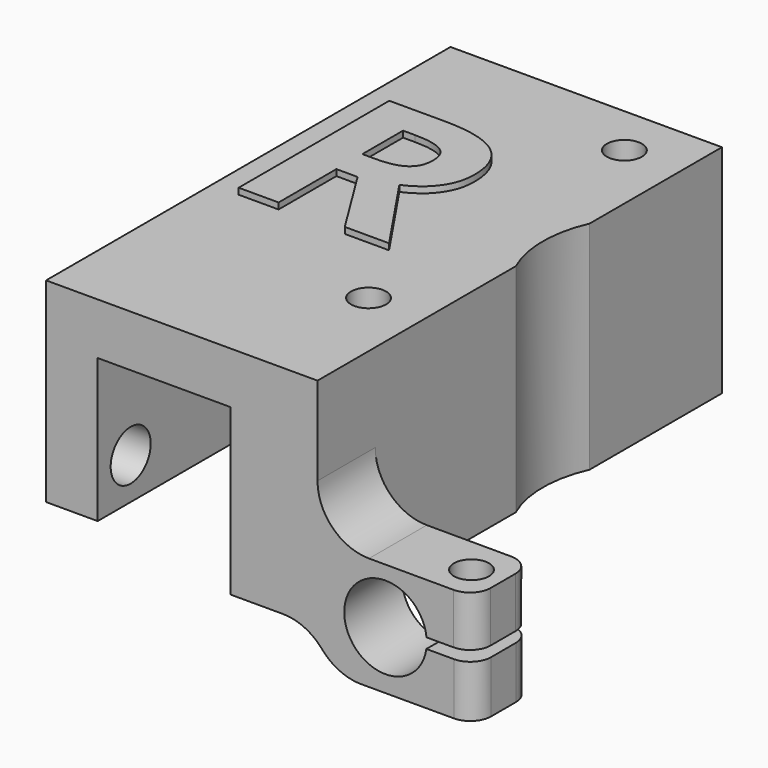
from build123d import *

# Parameters (mm, degrees)
F1_DEPTH      = 7
F2_DEPTH      = 42
F3_R          = 1.7
F3_R_2        = 11
F4_DEPTH      = 21.001
F5_R          = 4
F6_DEPTH      = 10
F7_DEPTH      = 21.001
F8_R          = 1.4
F9_DEPTH      = 11.021861364
F8_R_2        = 1.7
F10_DEPTH     = 4.9110969969
F11_R         = 5
F12_R         = 5
F13_R         = 5
F14_R         = 2
F15_R         = 2.2
F15_R_2       = 2.4255023423
F16_DEPTH     = 6
F17_TEXT_SIZE = 25.5631890872
F18_DEPTH     = 0.6


# Not quite as in the source:
# - a feature names something its author has since deleted; it is built from what else it names
# - Text() gives the source's letters only with a copy of the font that has no kerning and outlines rounded to 1/6400 em; it was checked with that copy


with BuildPart() as f1:
    # F0 (on Front) → F1 (new body)
    with BuildSketch(Plane.XZ):
        Polygon((-18.6721007523, 29.8099789735), (-18.6721007523, 10.8925135386), (-13.6721007523, 10.8925135386), (-13.6721007523, 24.8099789735), (-0.7721007523, 24.8099789735), (-0.7721007523, 8.8099789735), (7.6380548998, 8.8099789735), (7.6380548998, 16.2656020473), (7.6380548998, 29.8099789735), align=None)
        Polygon((22.8263195603, 16.2417280634), (7.6380548998, 16.2656020473), (7.6380548998, 8.8099789735), (9.0533044869, 5.2860832236), (22.8553367778, 5.2860832236), (22.8553367778, 10.343908232), (16.1860510706, 10.343908232), (16.1860510706, 11.3388913612), (22.8263195603, 11.3388913612), align=None)
    extrude(amount=F1_DEPTH)

    # F0 (on Front) → F2 (join)
    with BuildSketch(Plane.XZ):
        Polygon((-18.6721007523, 29.8099789735), (-18.6721007523, 10.8925135386), (-13.6721007523, 10.8925135386), (-13.6721007523, 24.8099789735), (-0.7721007523, 24.8099789735), (-0.7721007523, 8.8099789735), (7.6380548998, 8.8099789735), (7.6380548998, 16.2656020473), (7.6380548998, 29.8099789735), align=None)
    extrude(amount=-F2_DEPTH)

    # F3 (on face) → F4 (cut, through all)
    with BuildSketch(Plane(origin=(0, 0, 8.8099789735), x_dir=(1, 0, 0), z_dir=(0, 0, -1))):
        with Locations((2.1850741468, -6)):
            Circle(F3_R)
        with Locations((2.1850741468, -37)):
            Circle(F3_R)
        with Locations((17.6850741468, -21.5)):
            Circle(F3_R_2)
    extrude(amount=-F4_DEPTH, mode=Mode.SUBTRACT)

    # F5 (on face) → F6 (cut)
    with BuildSketch(Plane.XZ.offset(7)):
        with Locations((14.2278992477, 10.8989789735)):
            Circle(F5_R)
    extrude(amount=-F6_DEPTH, mode=Mode.SUBTRACT)

    # F3 (on face) → F7 (cut, through all)
    with BuildSketch(Plane(origin=(0, 0, 8.8099789735), x_dir=(1, 0, 0), z_dir=(0, 0, -1))):
        with Locations((2.1850741468, -6)):
            Circle(F3_R)
        with Locations((2.1850741468, -37)):
            Circle(F3_R)
        with Locations((17.6850741468, -21.5)):
            Circle(F3_R_2)
    extrude(amount=-F7_DEPTH, mode=Mode.SUBTRACT)

    # F8 (on face) → F9 (cut, through all)
    with BuildSketch(Plane(origin=(0.0255862274, 0, 16.2775678616), x_dir=(0.9999987646, 0, -0.0015718685), z_dir=(0.0015718685, 0, 0.9999987646))):
        with Locations((19.8007615007, -3.5767070949)):
            Circle(F8_R)
    extrude(amount=-F9_DEPTH, mode=Mode.SUBTRACT)

    # F8 (on face) → F10 (cut, through all)
    with BuildSketch(Plane(origin=(0.0255862274, 0, 16.2775678616), x_dir=(0.9999987646, 0, -0.0015718685), z_dir=(0.0015718685, 0, 0.9999987646))):
        with Locations((19.8007615007, -3.5767070949)):
            Circle(F8_R_2)
        with Locations((19.8007615007, -3.5767070949)):
            Circle(F8_R, mode=Mode.SUBTRACT)
    extrude(amount=-F10_DEPTH, mode=Mode.SUBTRACT)

    # F11
    f11_edges = [f1.edges().sort_by_distance(p)[0] for p in [
        (7.638055, -3.5, 16.265602),
    ]]
    fillet(f11_edges, radius=F11_R)

    # F12
    f12_edges = [f1.edges().sort_by_distance(p)[0] for p in [
        (7.638055, -3.5, 8.809979),
    ]]
    fillet(f12_edges, radius=F12_R)

    # F13
    f13_edges = [f1.edges().sort_by_distance(p)[0] for p in [
        (9.053304, -3.5, 5.286083),
    ]]
    fillet(f13_edges, radius=F13_R)

    # F14
    f14_edges = [f1.edges().sort_by_distance(p)[0] for p in [
        (22.82632, -7, 13.79031),
        (22.855337, -7, 7.814996),
        (22.82632, 0, 13.79031),
        (22.855337, 0, 7.814996),
    ]]
    fillet(f14_edges, radius=F14_R)

    # F15 (on face) → F16 (cut)
    with BuildSketch(Plane(origin=(-18.6721007523, 0, 0), x_dir=(0, -1, 0), z_dir=(-1, 0, 0))):
        with Locations((-38, 14.8925135386)):
            Circle(F15_R)
        with Locations((3, 14.8925135386)):
            Circle(F15_R_2)
    extrude(amount=-F16_DEPTH, mode=Mode.SUBTRACT)

    # F17 (on face) → F18 (join)
    with BuildSketch(Plane.XY.offset(29.8099789735)):
        with Locations((-18.3553399984, 13.0669334903)):
            Text('R', F17_TEXT_SIZE, font='Open Sans', font_style=FontStyle.BOLD, text_align=(TextAlign.LEFT, TextAlign.BOTTOM))
    extrude(amount=F18_DEPTH)


solid = f1.part
